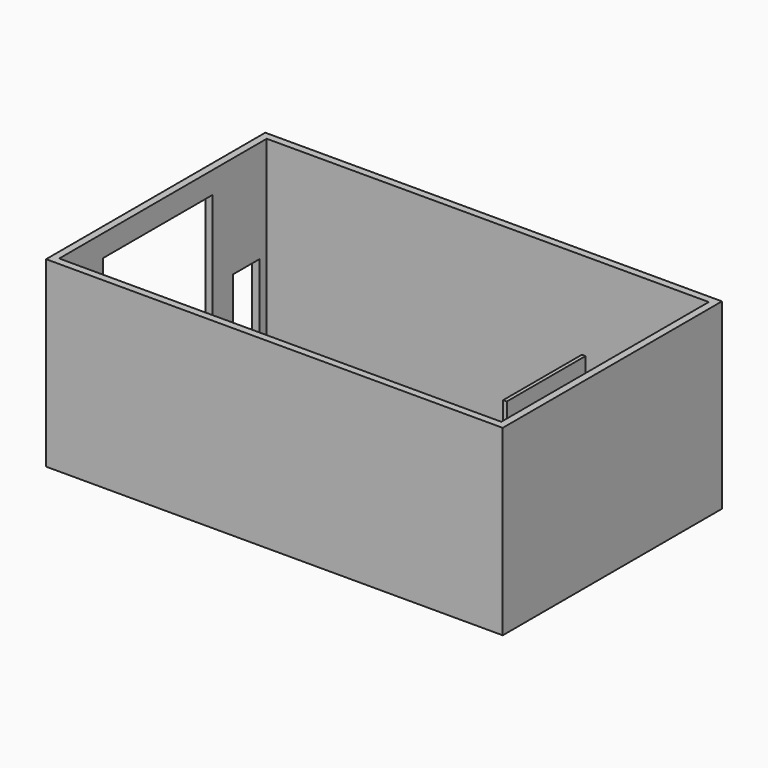
from build123d import *

# Parameters (mm, degrees)
F3_W      = 12700
F3_H      = 7620
F4_DEPTH  = 203.2
F5_W      = 12700
F5_H      = 7620
F5_W_2    = 12293.6
F5_H_2    = 7213.6
F6_DEPTH  = 4876.8
F7_W      = 3810
F7_H      = 4267.2
F7_W_2    = 914.4
F7_H_2    = 2032
F8_DEPTH  = 203.2
F9_W      = 457.2
F9_H      = 101.6
F10_DEPTH = 2438.4
F11_W     = 922.02
F11_H     = 2438.4
F12_DEPTH = 101.6


# Not quite as in the source:
# - a variable given as a bare number and used for a length is read in inches; the dataset says mm whatever the document's units were


with BuildPart() as f4:
    # F3 (on Top) → F4 (new body)
    with BuildSketch(Plane.XY):
        with Locations((1.8329881132, 153.9102016476)):
            Rectangle(F3_W, F3_H)
    extrude(amount=F4_DEPTH)

    # F5 (on face) → F6 (join)
    with BuildSketch(Plane.XY.offset(203.2)):
        with Locations((1.8329881132, 153.9102016476)):
            Rectangle(F5_W, F5_H)
        with Locations((1.8329881132, 153.9102016476)):
            Rectangle(F5_W_2, F5_H_2, mode=Mode.SUBTRACT)
    extrude(amount=F6_DEPTH)

    # F7 (on face) → F8 (cut, through all)
    with BuildSketch(Plane(origin=(-6348.1670118868, 0, 0), x_dir=(0, -1, 0), z_dir=(-1, 0, 0))):
        with Locations((23.8897983524, 2336.8)):
            Rectangle(F7_W, F7_H)
        with Locations((-3049.5102016476, 1219.2)):
            Rectangle(F7_W_2, F7_H_2)
    extrude(amount=-F8_DEPTH, mode=Mode.SUBTRACT)

    # F9 (on face) → F10 (join)
    with BuildSketch(Plane.XY.offset(203.2)):
        Polygon((2719.6329881132, -2081.2897983524), (2719.6329881132, 3760.7102016476), (2618.0329881132, 3760.7102016476), (2618.0329881132, -2182.8897983524), (4523.0329881132, -2182.8897983524), (4523.0329881132, -3452.8897983524), (4624.6329881132, -3452.8897983524), (4624.6329881132, -2182.8897983524), (4789.7329881132, -2182.8897983524), (4789.7329881132, -2081.2897983524), (4624.6329881132, -2081.2897983524), align=None)
        with Locations((5920.0329881132, -2132.0897983524)):
            Rectangle(F9_W, F9_H)
    extrude(amount=F10_DEPTH)

    # F11 (on face) → F12 (cut, through all)
    with BuildSketch(Plane(origin=(2618.0329881132, 0, 0), x_dir=(0, -1, 0), z_dir=(-1, 0, 0))):
        with Locations((-564.1202016476, 1422.4)):
            Rectangle(F11_W, F11_H)
    extrude(amount=-F12_DEPTH, mode=Mode.SUBTRACT)


solid = f4.part
